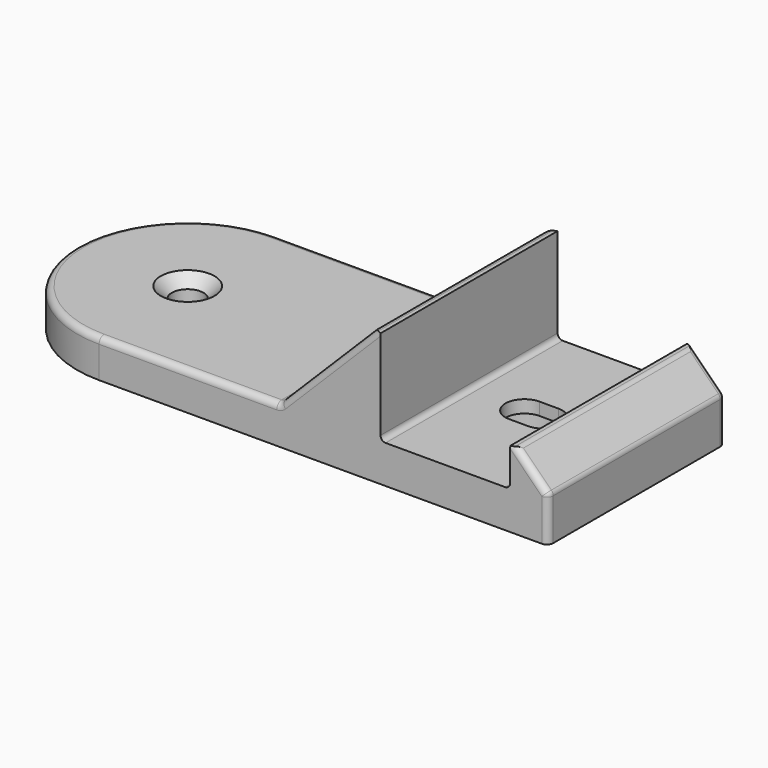
from build123d import *

# Parameters (mm, degrees)
F0_W            = 6
F0_H            = 35
F0_W_2          = 38.4963016563
F0_W_3          = 20.5
F1_DEPTH        = 6
F2_DEPTH        = 12
F3_SIZE         = 5
F4_DEPTH        = 21
F5_SIZE         = 5
F6_DEPTH        = 12
F7_T4_DEPTH     = 96.7203917112
F8_T1_DEPTH     = 35
F8_T3_DEPTH     = 28.0820880939
F8_T5_DEPTH     = 9.0857864376
F8_T7_DEPTH     = 9.1568542495
F8_T9_DEPTH     = 33
F8_T11_DEPTH    = 23.2989898732
F8_T13_DEPTH    = 37.0710678119
F8_T18_DEPTH    = 1.02
F8_T24_DEPTH    = 1.02
F8_T28_ANGLE    = 180
F8_T30_ANGLE    = 45
F8_T32_ANGLE    = 45
F9_R            = 0.8
F12_D           = 5
F12_CSINK_D     = 8.5
F12_CSINK_ANGLE = 90
F14_DEPTH       = 6
F15_DEPTH       = 4


# Not quite as in the source:
# - a fillet or chamfer that OpenCascade refuses, or shapes differently, is made with other operations: its cross-section is extruded or revolved along the edge and cut away or added


with BuildPart() as f1:
    # F0 (on Top) → F1 (new body)
    with BuildSketch(Plane.XY):
        with BuildLine():
            Line((-35.6485009767, -17.5), (-35.6485009767, 17.5))
            ThreePointArc((-35.6485009767, 17.5), (-53.1485009767, 0), (-35.6485009767, -17.5))
        make_face()
        with Locations((32.3478006796, 0)):
            Rectangle(F0_W, F0_H)
        with Locations((-16.4003501485, 0)):
            Rectangle(F0_W_2, F0_H)
        with Locations((19.0978006796, 0)):
            Rectangle(F0_W_3, F0_H)
        with Locations((5.8478006796, 0)):
            Rectangle(F0_W, F0_H)
    extrude(amount=F1_DEPTH)

    # F0 (on Top) → F2 (join)
    with BuildSketch(Plane.XY):
        with Locations((32.3478006796, 0)):
            Rectangle(F0_W, F0_H)
    extrude(amount=F2_DEPTH)

    # F3
    f3_edges = [f1.edges().sort_by_distance(p)[0] for p in [
        (35.347801, 0, 12),
    ]]
    chamfer(f3_edges, length=F3_SIZE)

    # F0 (on Top) → F4 (join)
    with BuildSketch(Plane.XY):
        with Locations((5.8478006796, 0)):
            Rectangle(F0_W, F0_H)
    extrude(amount=F4_DEPTH)

    # F5
    f5_edges = [f1.edges().sort_by_distance(p)[0] for p in [
        (2.847801, 0, 21),
    ]]
    chamfer(f5_edges, length=F5_SIZE)

    # F6 (add): a face of the model
    f6_faces = [f1.faces().sort_by_distance(p)[0] for p in [
        (2.8478006796, 0, 11),
    ]]
    extrude(f6_faces, amount=F6_DEPTH)

    # F7: chamfer of 12 on 4 edges, made by hand


with BuildPart() as f7_tool2:
    # F7_s3 → F7_t4 (new body)
    with BuildSketch(Plane.XZ.offset(-48.3601958556)):
        Polygon((2.8478006796, 16), (-9.1521993204, 4), (-9.1521993204, 16), align=None)
    extrude(amount=F7_T4_DEPTH)

    split(bisect_by=Plane.XY.offset(6), keep=Keep.TOP)


with BuildPart() as f1_1:
    add(f1.part)

    # F7_t1: cut F7_tool2
    add(f7_tool2.part, mode=Mode.SUBTRACT)

    # F8: fillet of radius 1 on 13 edges, made by hand

    # F8_s2 → F8_t1 (join)
    with BuildSketch(Plane.XZ.offset(-17.5)):
        with BuildLine():
            ThreePointArc((-7.5664128828, 6), (-7.1837294504, 6.0761204675), (-6.8593061016, 6.2928932188))
            Line((-6.8593061016, 6.2928932188), (-7.1521993204, 6))
            Line((-7.1521993204, 6), (-7.5664128828, 6))
        make_face()
    extrude(amount=F8_T1_DEPTH)

    # F8_s4 → F8_t3 (cut)
    with BuildSketch(Plane.YZ.offset(-35.6485009767)):
        with BuildLine():
            ThreePointArc((-16.5, 6), (-17.2071067812, 5.7071067812), (-17.5, 5))
            Line((-17.5, 5), (-17.5, 6))
            Line((-17.5, 6), (-16.5, 6))
        make_face()
        with BuildLine():
            ThreePointArc((17.5, 5), (17.2071067812, 5.7071067812), (16.5, 6))
            Line((16.5, 6), (17.5, 6))
            Line((17.5, 6), (17.5, 5))
        make_face()
    extrude(amount=F8_T3_DEPTH, mode=Mode.SUBTRACT)

    # F8_s6 → F8_t5 (cut)
    with BuildSketch(Plane.XY.offset(-2.5)):
        with BuildLine():
            ThreePointArc((35.3478006796, -16.5), (35.0549074608, -17.2071067812), (34.3478006796, -17.5))
            Line((34.3478006796, -17.5), (35.3478006796, -17.5))
            Line((35.3478006796, -17.5), (35.3478006796, -16.5))
        make_face()
        with BuildLine():
            ThreePointArc((34.3478006796, 17.5), (35.0549074608, 17.2071067812), (35.3478006796, 16.5))
            Line((35.3478006796, 16.5), (35.3478006796, 17.5))
            Line((35.3478006796, 17.5), (34.3478006796, 17.5))
        make_face()
    extrude(amount=F8_T5_DEPTH, mode=Mode.SUBTRACT)

    # F8_s8 → F8_t7 (cut)
    with BuildSketch(Plane(origin=(7.4061333868, 0, -7.4061333868), x_dir=(0, 1, 0), z_dir=(0.7071067812, 0, -0.7071067812))):
        with BuildLine():
            ThreePointArc((-16.5, 29.9444170289), (-17.2071067812, 29.6515238101), (-17.5, 28.9444170289))
            Line((-17.5, 28.9444170289), (-17.5, 29.9444170289))
            Line((-17.5, 29.9444170289), (-16.5, 29.9444170289))
        make_face()
        with BuildLine():
            ThreePointArc((17.5, 28.9444170289), (17.2071067812, 29.6515238101), (16.5, 29.9444170289))
            Line((16.5, 29.9444170289), (17.5, 29.9444170289))
            Line((17.5, 29.9444170289), (17.5, 28.9444170289))
        make_face()
    extrude(amount=F8_T7_DEPTH, mode=Mode.SUBTRACT)

    # F8_s10 → F8_t9 (cut)
    with BuildSketch(Plane.XZ.offset(-16.5)):
        with BuildLine():
            ThreePointArc((35.3478006796, 6.5857864376), (35.2716802121, 6.96846987), (35.0549074608, 7.2928932188))
            Line((35.0549074608, 7.2928932188), (35.3478006796, 7))
            Line((35.3478006796, 7), (35.3478006796, 6.5857864376))
        make_face()
    extrude(amount=F8_T9_DEPTH, mode=Mode.SUBTRACT)

    # F8_s12 → F8_t11 (cut)
    with BuildSketch(Plane(origin=(-0.2832064414, 0, -0.2832064414), x_dir=(0, 1, 0), z_dir=(0.7071067812, 0, 0.7071067812))):
        with BuildLine():
            ThreePointArc((17.5, 8.300009327), (17.2071067812, 9.0071161082), (16.5, 9.300009327))
            Line((16.5, 9.300009327), (17.5, 9.300009327))
            Line((17.5, 9.300009327), (17.5, 8.300009327))
        make_face()
        with BuildLine():
            ThreePointArc((-16.5, 9.300009327), (-17.2071067812, 9.0071161082), (-17.5, 8.300009327))
            Line((-17.5, 8.300009327), (-17.5, 9.300009327))
            Line((-17.5, 9.300009327), (-16.5, 9.300009327))
        make_face()
    extrude(amount=F8_T11_DEPTH, mode=Mode.SUBTRACT)

    # F8_s14 → F8_t13 (cut)
    with BuildSketch(Plane.XZ.offset(-18.5355339059)):
        with BuildLine():
            ThreePointArc((30.6406938984, 11.7071067812), (30.3162705496, 11.9238795325), (29.9335871172, 12))
            Line((29.9335871172, 12), (30.3478006796, 12))
            Line((30.3478006796, 12), (30.6406938984, 11.7071067812))
        make_face()
        with BuildLine():
            ThreePointArc((8.262014242, 21), (7.8793308096, 20.9238795325), (7.5549074608, 20.7071067812))
            Line((7.5549074608, 20.7071067812), (7.8478006796, 21))
            Line((7.8478006796, 21), (8.262014242, 21))
        make_face()
    extrude(amount=F8_T13_DEPTH, mode=Mode.SUBTRACT)


with BuildPart() as f8_tool16:
    # F8_s17 → F8_t18 (new body)
    with BuildSketch(Plane.XZ.offset(16.5)):
        Polygon((34.3478006796, 6.5857864376), (35.3678006796, 6.5857864376), (35.3678006796, 7.0082842712), (35.0690495964, 7.3070353544), align=None)
    extrude(amount=F8_T18_DEPTH)

    # F8_s19 → F8_t20 (revolve, cut)
    with BuildSketch(Plane(origin=(34.3478006796, -16.5, 6.5857864376), x_dir=(-0.9238795325, 0, -0.3826834324), z_dir=(-0.3826834324, 0, 0.9238795325))):
        with BuildLine():
            ThreePointArc((0, -1), (1, 0), (0, 1))
            Line((0, 1), (0, -1))
        make_face()
    revolve(axis=Axis((34.3478006796, -16.5, 6.5857864376), (0, -1, 0)), mode=Mode.SUBTRACT)


with BuildPart() as f1_2:
    add(f1_1.part)

    # F8_t15: cut F8_tool16
    add(f8_tool16.part, mode=Mode.SUBTRACT)


with BuildPart() as f8_tool22:
    # F8_s23 → F8_t24 (new body)
    with BuildSketch(Plane.XZ.offset(-16.5)):
        Polygon((34.3478006796, 6.5857864376), (35.3678006796, 6.5857864376), (35.3678006796, 7.0082842712), (35.0690495964, 7.3070353544), align=None)
    extrude(amount=-F8_T24_DEPTH)

    # F8_s25 → F8_t26 (revolve, cut)
    with BuildSketch(Plane(origin=(34.3478006796, 16.5, 6.5857864376), x_dir=(-0.9238795325, 0, -0.3826834324), z_dir=(0.3826834324, 0, -0.9238795325))):
        with BuildLine():
            ThreePointArc((0, -1), (1, 0), (0, 1))
            Line((0, 1), (0, -1))
        make_face()
    revolve(axis=Axis((34.3478006796, 16.5, 6.5857864376), (0, 1, 0)), mode=Mode.SUBTRACT)


with BuildPart() as f1_3:
    add(f1_2.part)

    # F8_t21: cut F8_tool22
    add(f8_tool22.part, mode=Mode.SUBTRACT)

    # F8_s27 → F8_t28 (revolve, cut)
    with BuildSketch(Plane.YZ.offset(-35.6485009767)):
        with BuildLine():
            ThreePointArc((16.5, 6), (17.2071067812, 5.7071067812), (17.5, 5))
            Line((17.5, 5), (17.5, 6))
            Line((17.5, 6), (16.5, 6))
        make_face()
    revolve(axis=Axis((-35.6485009767, 0, 6), (0, 0, 1)), revolution_arc=F8_T28_ANGLE, mode=Mode.SUBTRACT)

    # F8_s29 → F8_t30 (revolve, cut)
    with BuildSketch(Plane.YZ.offset(-7.5664128828)):
        with BuildLine():
            ThreePointArc((-17.5, 5), (-17.2071067812, 5.7071067812), (-16.5, 6))
            Line((-16.5, 6), (-17.5, 6))
            Line((-17.5, 6), (-17.5, 5))
        make_face()
    revolve(axis=Axis((-7.5664128828, -17.5, 7), (0, -1, 0)), revolution_arc=F8_T30_ANGLE, mode=Mode.SUBTRACT)

    # F8_s31 → F8_t32 (revolve, cut)
    with BuildSketch(Plane.YZ.offset(-7.5664128828)):
        with BuildLine():
            ThreePointArc((17.5, 5), (17.2071067812, 5.7071067812), (16.5, 6))
            Line((16.5, 6), (17.5, 6))
            Line((17.5, 6), (17.5, 5))
        make_face()
    revolve(axis=Axis((-7.5664128828, 17.5, 7), (0, -1, 0)), revolution_arc=F8_T32_ANGLE, mode=Mode.SUBTRACT)

    # F9
    f9_edges = [f1_3.edges().sort_by_distance(p)[0] for p in [
        (8.847801, 0, 6),
        (29.347801, 0, 6),
    ]]
    fillet(f9_edges, radius=F9_R)

    # F12 (through all)
    with Locations(Plane.XY.offset(6)):
        with Locations((-35.6485009767, 0)):
            CounterSinkHole(F12_D / 2, F12_CSINK_D / 2, counter_sink_angle=F12_CSINK_ANGLE)

    # F13 (on face) → F14 (cut, through all)
    with BuildSketch(Plane.XY):
        with BuildLine():
            ThreePointArc((20.5978006796, -3), (23.5978006796, 0), (20.5978006796, 3))
            Line((20.5978006796, 3), (17.5978006796, 3))
            ThreePointArc((17.5978006796, 3), (14.5978006796, 0), (17.5978006796, -3))
            Line((17.5978006796, -3), (20.5978006796, -3))
        make_face()
    extrude(amount=F14_DEPTH, mode=Mode.SUBTRACT)

    # F13 (on face) → F15 (cut)
    with BuildSketch(Plane.XY):
        with BuildLine():
            ThreePointArc((20.5978006796, -6.25), (26.8478006796, 0), (20.5978006796, 6.25))
            Line((20.5978006796, 6.25), (17.5978006796, 6.25))
            ThreePointArc((17.5978006796, 6.25), (11.3478006796, 0), (17.5978006796, -6.25))
            Line((17.5978006796, -6.25), (20.5978006796, -6.25))
        make_face()
        with BuildLine():
            Line((17.5978006796, 3), (20.5978006796, 3))
            ThreePointArc((20.5978006796, 3), (23.5978006796, 0), (20.5978006796, -3))
            Line((20.5978006796, -3), (17.5978006796, -3))
            ThreePointArc((17.5978006796, -3), (14.5978006796, 0), (17.5978006796, 3))
        make_face(mode=Mode.SUBTRACT)
    extrude(amount=F15_DEPTH, mode=Mode.SUBTRACT)


solid = f1_3.part
